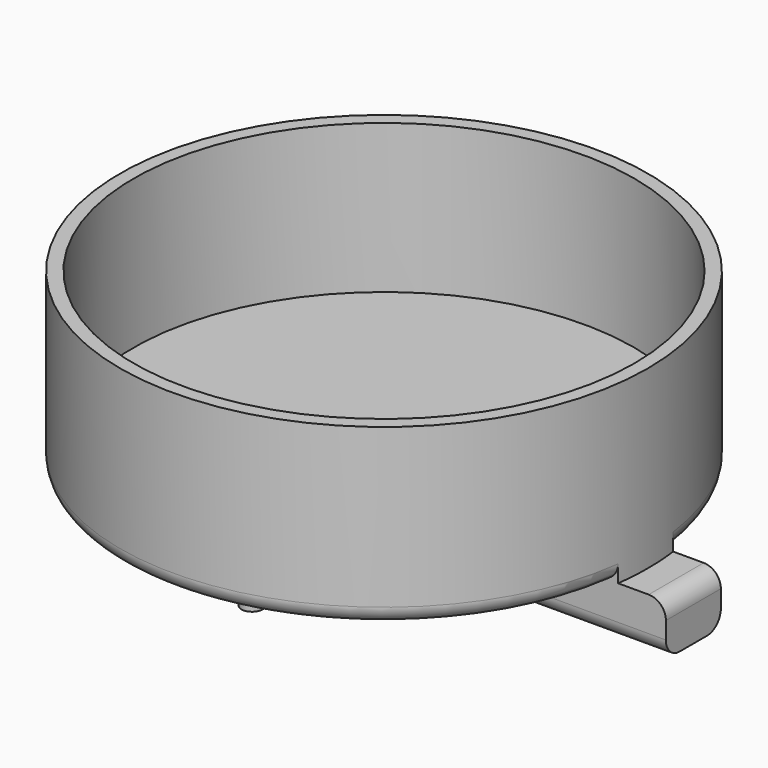
from build123d import *

# Parameters (mm, degrees)
F0_R         = 19.5
F1_DEPTH     = 13
F2_R         = 18.5
F3_DEPTH     = 11
F4_W         = 45.72
F4_H         = 5.08
F5_DEPTH     = 3.81
F6_T1_DEPTH  = 52.07
F6_T3_DEPTH  = 11.43
F6_T8_ANGLE  = 183.7142551891
F6_T13_ANGLE = 183.7142551891
F7_R         = 0.7920917612
F8_DEPTH     = 3.81


# Not quite as in the source:
# - a fillet or chamfer that OpenCascade refuses, or shapes differently, is made with other operations: its cross-section is extruded or revolved along the edge and cut away or added


with BuildPart() as f1:
    # F0 (on Top) → F1 (new body)
    with BuildSketch(Plane.XY):
        Circle(F0_R)
    extrude(amount=F1_DEPTH)

    # F2 (on face) → F3 (cut)
    with BuildSketch(Plane.XY.offset(13)):
        Circle(F2_R)
    extrude(amount=-F3_DEPTH, mode=Mode.SUBTRACT)

    # F4 (on face) → F5 (join)
    with BuildSketch(Plane(origin=(0, 0, 0), x_dir=(1, 0, 0), z_dir=(0, 0, -1))):
        Rectangle(F4_W, F4_H)
    extrude(amount=F5_DEPTH)

    # F6: fillet of radius 1.27 on 6 edges, made by hand

    # F6_s2 → F6_t1 (cut)
    with BuildSketch(Plane.YZ.offset(-26.035)):
        with BuildLine():
            ThreePointArc((-2.54, -2.54), (-2.1680256121, -3.4380256121), (-1.27, -3.81))
            Line((-1.27, -3.81), (-2.54, -3.81))
            Line((-2.54, -3.81), (-2.54, -2.54))
        make_face()
        with BuildLine():
            ThreePointArc((2.54, -2.54), (2.1680256121, -3.4380256121), (1.27, -3.81))
            Line((1.27, -3.81), (2.54, -3.81))
            Line((2.54, -3.81), (2.54, -2.54))
        make_face()
    extrude(amount=F6_T1_DEPTH, mode=Mode.SUBTRACT)

    # F6_s4 → F6_t3 (cut)
    with BuildSketch(Plane.XZ.offset(-5.715)):
        with BuildLine():
            ThreePointArc((-21.59, 0), (-22.4880256121, -0.3719743879), (-22.86, -1.27))
            Line((-22.86, -1.27), (-22.86, 0))
            Line((-22.86, 0), (-21.59, 0))
        make_face()
        with BuildLine():
            ThreePointArc((21.59, 0), (22.4880256121, -0.3719743879), (22.86, -1.27))
            Line((22.86, -1.27), (22.86, 0))
            Line((22.86, 0), (21.59, 0))
        make_face()
    extrude(amount=F6_T3_DEPTH, mode=Mode.SUBTRACT)


with BuildPart() as f6_tool6:
    # F6_s7 → F6_t8 (revolve)
    with BuildSketch(Plane(origin=(0, 0, 0), x_dir=(0, 0, 1), z_dir=(-0.0324073159, -0.999474745, 0))):
        with BuildLine():
            ThreePointArc((1.27, -19.5), (0.3719743879, -19.1280256121), (0, -18.23))
            Line((0, -18.23), (0, -19.5))
            Line((0, -19.5), (1.27, -19.5))
        make_face()
    revolve(axis=Axis((0, 0, 0), (0, 0, 1)), revolution_arc=F6_T8_ANGLE)

    split(bisect_by=Plane.XZ.offset(-2.54), keep=Keep.BOTTOM)


with BuildPart() as f1_1:
    add(f1.part)

    # F6_t5: cut F6_tool6
    add(f6_tool6.part, mode=Mode.SUBTRACT)


with BuildPart() as f6_tool11:
    # F6_s12 → F6_t13 (revolve)
    with BuildSketch(Plane(origin=(0, 0, 0), x_dir=(0, 0, 1), z_dir=(0.0324073159, 0.999474745, 0))):
        with BuildLine():
            ThreePointArc((1.27, -19.5), (0.3719743879, -19.1280256121), (0, -18.23))
            Line((0, -18.23), (0, -19.5))
            Line((0, -19.5), (1.27, -19.5))
        make_face()
    revolve(axis=Axis((0, 0, 0), (0, 0, 1)), revolution_arc=F6_T13_ANGLE)

    split(bisect_by=Plane.XZ.offset(2.54), keep=Keep.TOP)


with BuildPart() as f1_2:
    add(f1_1.part)

    # F6_t10: cut F6_tool11
    add(f6_tool11.part, mode=Mode.SUBTRACT)

    # F7 (on face) → F8 (join, through all)
    with BuildSketch(Plane(origin=(0, 0, 0), x_dir=(1, 0, 0), z_dir=(0, 0, -1))):
        with Locations((10.5457008786, -6.0885632411)):
            Circle(F7_R)
        with Locations((-10.5457008786, -6.0885632411)):
            Circle(F7_R)
        with Locations((0, 12.1771264821)):
            Circle(F7_R)
    extrude(amount=F8_DEPTH)


solid = f1_2.part
